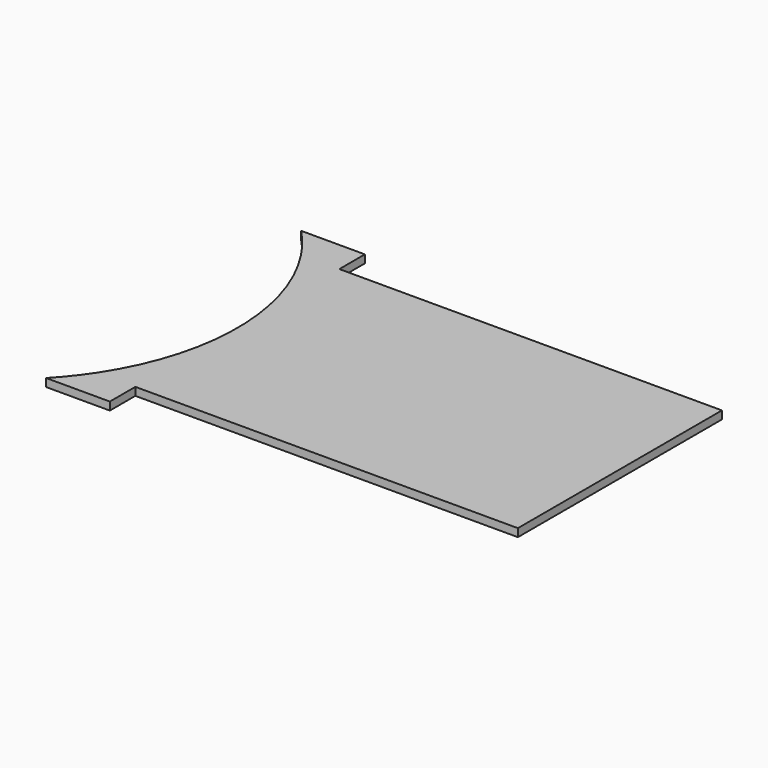
from build123d import *

# Parameters (mm, degrees)
F0_W     = 25.4
F0_H     = 3.175
F1_DEPTH = 3.175
F6_DEPTH = 3.176


# Not quite as in the source:
# - the program builds the solid bodies; features that only make, move or delete a surface that nothing else refers to are left out


with BuildPart() as f1:
    # F0 (on Top) → F1 (new body)
    with BuildSketch(Plane.XY):
        with BuildLine():
            Line((-120.0661680937, 14.7140049219), (-109.9481630411, 14.7140049219))
            ThreePointArc((-109.9481630411, 14.7140049219), (-114.7266583166, 21.2874831724), (-120.0661680937, 27.4140049219))
            Line((-120.0661680937, 27.4140049219), (-120.0661680937, 14.7140049219))
        make_face()
        with BuildLine():
            ThreePointArc((-109.9481630411, -86.8859950781), (-94.6661680937, -36.0859950781), (-109.9481630411, 14.7140049219))
            Line((-109.9481630411, 14.7140049219), (-120.0661680937, 14.7140049219))
            Line((-120.0661680937, 14.7140049219), (-120.0661680937, -86.8859950781))
            Line((-120.0661680937, -86.8859950781), (-109.9481630411, -86.8859950781))
        make_face()
        with Locations((32.3338319063, 13.1265049219)):
            Rectangle(F0_W, F0_H)
        with BuildLine():
            Line((-94.6661680937, -86.8859950781), (-109.9481630411, -86.8859950781))
            ThreePointArc((-109.9481630411, -86.8859950781), (-114.7266583166, -93.4594733286), (-120.0661680937, -99.5859950781))
            Line((-120.0661680937, -99.5859950781), (-94.6661680937, -99.5859950781))
            Line((-94.6661680937, -99.5859950781), (-94.6661680937, -86.8859950781))
        make_face()
        with BuildLine():
            Line((-89.0957787633, 14.7140049219), (-94.6661680937, 14.7140049219))
            Line((-94.6661680937, 14.7140049219), (-109.9481630411, 14.7140049219))
            ThreePointArc((-109.9481630411, 14.7140049219), (-94.6661680937, -36.0859950781), (-109.9481630411, -86.8859950781))
            Line((-109.9481630411, -86.8859950781), (-94.6661680937, -86.8859950781))
            Line((-94.6661680937, -86.8859950781), (19.6338319063, -86.8859950781))
            Line((19.6338319063, -86.8859950781), (19.6338319063, -83.7109950781))
            Line((19.6338319063, -83.7109950781), (45.0338319063, -83.7109950781))
            Line((45.0338319063, -83.7109950781), (45.0338319063, -86.8859950781))
            Line((45.0338319063, -86.8859950781), (57.7338319063, -86.8859950781))
            Line((57.7338319063, -86.8859950781), (57.7338319063, 14.7140049219))
            Line((57.7338319063, 14.7140049219), (45.0338319063, 14.7140049219))
            Line((45.0338319063, 14.7140049219), (45.0338319063, 11.5390049219))
            Line((45.0338319063, 11.5390049219), (19.6338319063, 11.5390049219))
            Line((19.6338319063, 11.5390049219), (19.6338319063, 14.7140049219))
            Line((19.6338319063, 14.7140049219), (-89.0957787633, 14.7140049219))
        make_face()
        with Locations((32.3338319063, -85.2984950781)):
            Rectangle(F0_W, F0_H)
        with BuildLine():
            ThreePointArc((-120.0661680937, -99.5859950781), (-114.7266583166, -93.4594733286), (-109.9481630411, -86.8859950781))
            Line((-109.9481630411, -86.8859950781), (-120.0661680937, -86.8859950781))
            Line((-120.0661680937, -86.8859950781), (-120.0661680937, -99.5859950781))
        make_face()
        with BuildLine():
            Line((-109.9481630411, 14.7140049219), (-94.6661680937, 14.7140049219))
            Line((-94.6661680937, 14.7140049219), (-94.6661680937, 27.4140049219))
            Line((-94.6661680937, 27.4140049219), (-120.0661680937, 27.4140049219))
            ThreePointArc((-120.0661680937, 27.4140049219), (-114.7266583166, 21.2874831724), (-109.9481630411, 14.7140049219))
        make_face()
    extrude(amount=F1_DEPTH)

    # F0 (on Top) → F6 (cut, through all)
    with BuildSketch(Plane.XY):
        with BuildLine():
            ThreePointArc((-109.9481630411, -86.8859950781), (-94.6661680937, -36.0859950781), (-109.9481630411, 14.7140049219))
            Line((-109.9481630411, 14.7140049219), (-120.0661680937, 14.7140049219))
            Line((-120.0661680937, 14.7140049219), (-120.0661680937, -86.8859950781))
            Line((-120.0661680937, -86.8859950781), (-109.9481630411, -86.8859950781))
        make_face()
        with BuildLine():
            Line((-120.0661680937, 14.7140049219), (-109.9481630411, 14.7140049219))
            ThreePointArc((-109.9481630411, 14.7140049219), (-114.7266583166, 21.2874831724), (-120.0661680937, 27.4140049219))
            Line((-120.0661680937, 27.4140049219), (-120.0661680937, 14.7140049219))
        make_face()
        with BuildLine():
            ThreePointArc((-120.0661680937, -99.5859950781), (-114.7266583166, -93.4594733286), (-109.9481630411, -86.8859950781))
            Line((-109.9481630411, -86.8859950781), (-120.0661680937, -86.8859950781))
            Line((-120.0661680937, -86.8859950781), (-120.0661680937, -99.5859950781))
        make_face()
    extrude(amount=F6_DEPTH, mode=Mode.SUBTRACT)


solid = f1.part
